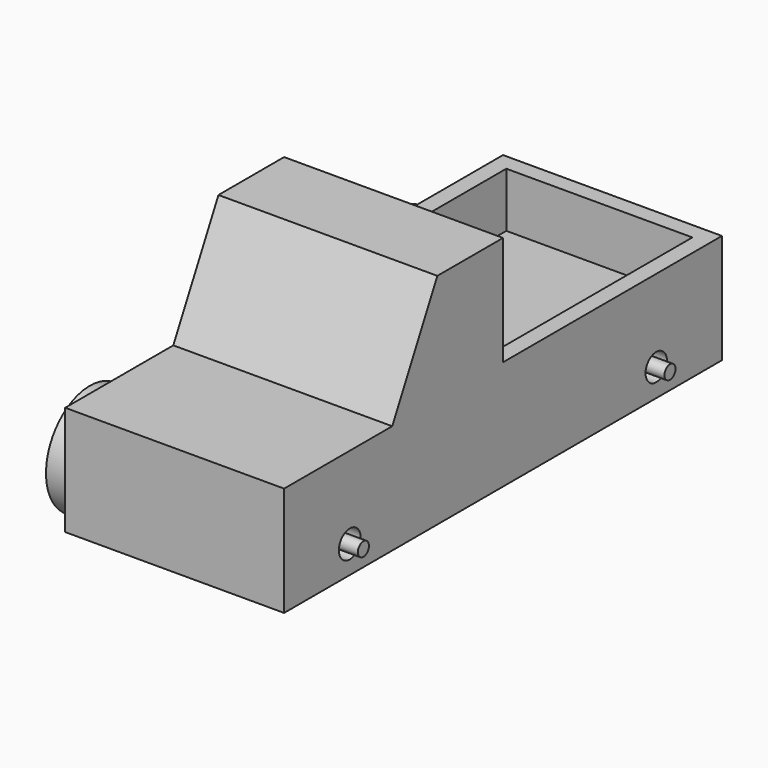
from build123d import *

# Parameters (mm, degrees)
F0_W      = 100
F0_H      = 20
F1_DEPTH  = 40
F5_R      = 2.5
F5_R_2    = 2.444231729
F6_DEPTH  = 40.0010001
F7_W      = 34
F7_H      = 44
F8_DEPTH  = 10
F9_R      = 1.2598965516
F10_DEPTH = 42.5
F11_DEPTH = 2.5
F12_R     = 10
F13_DEPTH = 5


# Not quite as in the source:
# - a feature of the source that left no trace in its solid (it failed there, or was rolled back) is left out
# - the program builds the solid bodies; features that only make, move or delete a surface that nothing else refers to are left out


with BuildPart() as f1:
    # F0 (on Right) → F1 (new body)
    with BuildSketch(Plane.YZ):
        Rectangle(F0_W, F0_H)
    extrude(amount=F1_DEPTH)

    # F3 (on face) → F4 section 0
    with BuildSketch(Plane(origin=(0, 0, 0), x_dir=(0, -1, 0), z_dir=(-1, 0, 0))):
        Polygon((0, 30), (0, 10), (25.307764064, 10), (15, 30), align=None)
    # F2 (on face) → F4 section 1
    with BuildSketch(Plane.YZ.offset(40)):
        Polygon((-25.307764064, 10), (0, 10), (0, 30), (-15, 30), align=None)
    loft()

    # F5 (on face) → F6 (cut, through all)
    with BuildSketch(Plane.YZ.offset(40)):
        with Locations((-35, -5)):
            Circle(F5_R)
        with Locations((35, -5)):
            Circle(F5_R_2)
    extrude(amount=-F6_DEPTH, mode=Mode.SUBTRACT)

    # F7 (on face) → F8 (cut)
    with BuildSketch(Plane.XY.offset(10)):
        with Locations((20, 25)):
            Rectangle(F7_W, F7_H)
    extrude(amount=-F8_DEPTH, mode=Mode.SUBTRACT)


with BuildPart() as f10:
    # F9 (on Right) → F10 (new body)
    with BuildSketch(Plane.YZ):
        with Locations((35.0127312975, -4.9924484168)):
            Circle(F9_R)
    extrude(amount=F10_DEPTH)

    # F9 (on Right) → F11 (join)
    with BuildSketch(Plane.YZ):
        with Locations((35.0127312975, -4.9924484168)):
            Circle(F9_R)
    extrude(amount=-F11_DEPTH)

    # F12 (on face) → F13 (join)
    with BuildSketch(Plane(origin=(-2.5, 0, 0), x_dir=(0, -1, 0), z_dir=(-1, 0, 0))):
        with Locations((-35.0127312975, -4.9924484168)):
            Circle(F12_R)
    extrude(amount=F13_DEPTH)


with BuildPart() as f14_1:
    # F14: instance of F10
    add(f10.part.mirror(Plane.XZ))


solid = Compound([f1.part, f10.part, f14_1.part])
